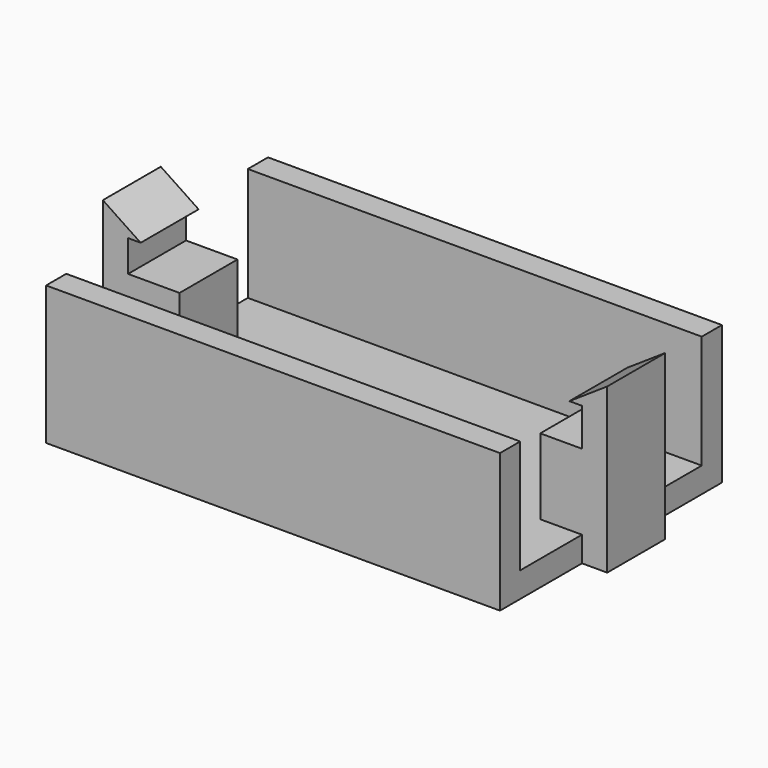
from build123d import *

# Parameters (mm, degrees)
F0_W      = 36
F0_H      = 2
F1_DEPTH  = 2
F0_W_2    = 4.0826744884
F0_H_2    = 5.745283328
F2_DEPTH  = 8.5
F3_DEPTH  = 11
F0_W_3    = 2
F4_DEPTH  = 11
F5_W      = 3
F5_H      = 5.745283328
F5_W_2    = 2
F5_W_3    = 1
F6_DEPTH  = 2
F8_DEPTH  = 5.745283328
F10_DEPTH = 5.745283328
F0_W_4    = 3.3082471341
F11_DEPTH = 8


# Not quite as in the source:
# - a feature names something its author has since deleted; it is built from what else it names


with BuildPart() as f1:
    # F0 (on Top) → F1 (new body)
    with BuildSketch(Plane.XY):
        with Locations((0, -10)):
            Rectangle(F0_W, F0_H)
        Polygon((-18, -9), (18, -9), (18, -2.872641664), (14.6917528659, -2.872641664), (14.6917528659, 2.872641664), (18, 2.872641664), (18, 9), (-18, 9), (-18, 2.872641664), (-13.9173255116, 2.872641664), (-13.9173255116, -2.872641664), (-18, -2.872641664), align=None)
    extrude(amount=F1_DEPTH)

    # F0 (on Top) → F2 (join)
    with BuildSketch(Plane.XY):
        with Locations((-15.9586627558, 0)):
            Rectangle(F0_W_2, F0_H_2)
    extrude(amount=F2_DEPTH)

    # F0 (on Top) → F3 (join)
    with BuildSketch(Plane.XY):
        with Locations((0, -10)):
            Rectangle(F0_W, F0_H)
        with Locations((0, 10)):
            Rectangle(F0_W, F0_H)
    extrude(amount=F3_DEPTH)

    # F0 (on Top) → F4 (join)
    with BuildSketch(Plane.XY):
        with Locations((-19, 0)):
            Rectangle(F0_W_3, F0_H_2)
        with Locations((19, 0)):
            Rectangle(F0_W_3, F0_H_2)
    extrude(amount=F4_DEPTH)

    # F5 (on face) → F6 (join)
    with BuildSketch(Plane.XY.offset(11)):
        with Locations((18.5, 0)):
            Rectangle(F5_W, F5_H)
        with Locations((-19, 0)):
            Rectangle(F5_W_2, F5_H)
        with Locations((-17.5, 0)):
            Rectangle(F5_W_3, F5_H)
    extrude(amount=F6_DEPTH)

    # F7 (on face) → F8 (cut, through all)
    with BuildSketch(Plane.XZ.offset(2.872641664)):
        Polygon((-20, 13), (-17, 11), (-17, 13), align=None)
    extrude(amount=-F8_DEPTH, mode=Mode.SUBTRACT)

    # F9 (on face) → F10 (cut, through all)
    with BuildSketch(Plane.XZ.offset(2.872641664)):
        Polygon((17, 13), (17, 11), (20, 13), align=None)
    extrude(amount=-F10_DEPTH, mode=Mode.SUBTRACT)

    # F0 (on Top) → F11 (join)
    with BuildSketch(Plane.XY):
        with Locations((16.345876433, 0)):
            Rectangle(F0_W_4, F0_H_2)
    extrude(amount=F11_DEPTH)


solid = f1.part
